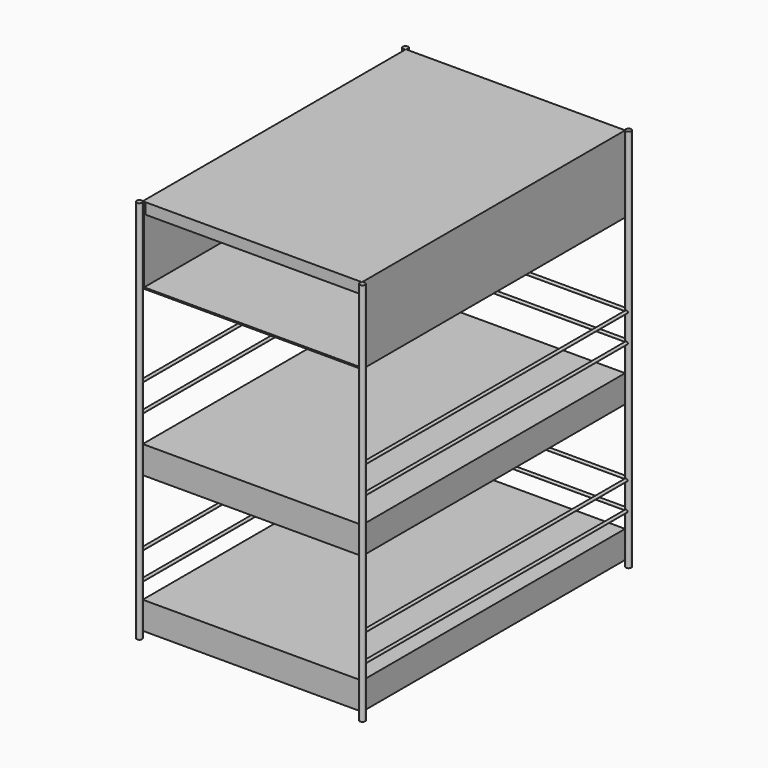
from build123d import *

# Parameters (mm, degrees)
F0_W      = 400
F0_H      = 140
F1_DEPTH  = 600
F0_H_2    = 50
F2_R      = 5
F3_DEPTH  = 701.04
F5_T      = -2.54
F4_W      = 390
F4_H      = 20
F6_DEPTH  = 25.4
F8_R      = 2.5
F9_DEPTH  = 607.822
F11_R     = 2.5
F12_DEPTH = 407.162


with BuildPart() as f1:
    # F0 (on Front) → F1 (new body)
    with BuildSketch(Plane.XZ):
        with Locations((0, 345)):
            Rectangle(F0_W, F0_H)
    extrude(amount=-F1_DEPTH)

    # F5
    f5_openings = [f1.faces().sort_by_distance(p)[0] for p in [
        (0, 0, 345),
    ]]
    offset(amount=F5_T, openings=f5_openings)

    # F4 (on face) → F6 (join)
    with BuildSketch(Plane.XZ):
        with Locations((0, 405)):
            Rectangle(F4_W, F4_H)
    extrude(amount=-F6_DEPTH)


with BuildPart() as f1b:
    # F0 (on Front) → F1, piece 2 (new body)
    with BuildSketch(Plane.XZ):
        Rectangle(F0_W, F0_H_2)
    extrude(amount=-F1_DEPTH)


with BuildPart() as f1c:
    # F0 (on Front) → F1, piece 3 (new body)
    with BuildSketch(Plane.XZ):
        with Locations((0, -250)):
            Rectangle(F0_W, F0_H_2)
    extrude(amount=-F1_DEPTH)


with BuildPart() as f3:
    # F2 (on face) → F3 (new body)
    with BuildSketch(Plane.XY.offset(415)):
        with Locations((203.5355339059, -3.5355339059)):
            Circle(F2_R)
    extrude(amount=-F3_DEPTH)


with BuildPart() as f3b:
    # F2 (on face) → F3, piece 2 (new body)
    with BuildSketch(Plane.XY.offset(415)):
        with Locations((203.5355339059, 603.5355339059)):
            Circle(F2_R)
    extrude(amount=-F3_DEPTH)


with BuildPart() as f3c:
    # F2 (on face) → F3, piece 3 (new body)
    with BuildSketch(Plane.XY.offset(415)):
        with Locations((-203.5355339059, 603.5355339059)):
            Circle(F2_R)
    extrude(amount=-F3_DEPTH)


with BuildPart() as f3d:
    # F2 (on face) → F3, piece 4 (new body)
    with BuildSketch(Plane.XY.offset(415)):
        with Locations((-202.7795129572, -4.156237207)):
            Circle(F2_R)
    extrude(amount=-F3_DEPTH)


with BuildPart() as f9:
    # F8 (on face) → F9 (new body)
    with BuildSketch(Plane(origin=(0, 603.5355339059, 0), x_dir=(-1, 0, 0), z_dir=(0, 1, 0))):
        with Locations((202.33258605, 125)):
            Circle(F8_R)
    extrude(amount=-F9_DEPTH)


with BuildPart() as f9b:
    # F8 (on face) → F9, piece 2 (new body)
    with BuildSketch(Plane(origin=(0, 603.5355339059, 0), x_dir=(-1, 0, 0), z_dir=(0, 1, 0))):
        with Locations((202.33258605, 75)):
            Circle(F8_R)
    extrude(amount=-F9_DEPTH)


with BuildPart() as f9c:
    # F8 (on face) → F9, piece 3 (new body)
    with BuildSketch(Plane(origin=(0, 603.5355339059, 0), x_dir=(-1, 0, 0), z_dir=(0, 1, 0))):
        with Locations((-203.3087313175, 125)):
            Circle(F8_R)
    extrude(amount=-F9_DEPTH)


with BuildPart() as f9d:
    # F8 (on face) → F9, piece 4 (new body)
    with BuildSketch(Plane(origin=(0, 603.5355339059, 0), x_dir=(-1, 0, 0), z_dir=(0, 1, 0))):
        with Locations((-203.3087313175, 75)):
            Circle(F8_R)
    extrude(amount=-F9_DEPTH)


with BuildPart() as f9e:
    # F8 (on face) → F9, piece 5 (new body)
    with BuildSketch(Plane(origin=(0, 603.5355339059, 0), x_dir=(-1, 0, 0), z_dir=(0, 1, 0))):
        with Locations((202.33258605, -145)):
            Circle(F8_R)
    extrude(amount=-F9_DEPTH)


with BuildPart() as f9f:
    # F8 (on face) → F9, piece 6 (new body)
    with BuildSketch(Plane(origin=(0, 603.5355339059, 0), x_dir=(-1, 0, 0), z_dir=(0, 1, 0))):
        with Locations((202.33258605, -195)):
            Circle(F8_R)
    extrude(amount=-F9_DEPTH)


with BuildPart() as f9g:
    # F8 (on face) → F9, piece 7 (new body)
    with BuildSketch(Plane(origin=(0, 603.5355339059, 0), x_dir=(-1, 0, 0), z_dir=(0, 1, 0))):
        with Locations((-202.9743790627, -145)):
            Circle(F8_R)
    extrude(amount=-F9_DEPTH)


with BuildPart() as f9h:
    # F8 (on face) → F9, piece 8 (new body)
    with BuildSketch(Plane(origin=(0, 603.5355339059, 0), x_dir=(-1, 0, 0), z_dir=(0, 1, 0))):
        with Locations((-202.9743790627, -195)):
            Circle(F8_R)
    extrude(amount=-F9_DEPTH)


with BuildPart() as f12:
    # F11 (on face) → F12 (new body)
    with BuildSketch(Plane.YZ.offset(-203.5355339059)):
        with Locations((604.149222374, 124.5824322104)):
            Circle(F11_R)
    extrude(amount=F12_DEPTH)


with BuildPart() as f12b:
    # F11 (on face) → F12, piece 2 (new body)
    with BuildSketch(Plane.YZ.offset(-203.5355339059)):
        with Locations((604.149222374, 75.2380788326)):
            Circle(F11_R)
    extrude(amount=F12_DEPTH)


with BuildPart() as f12c:
    # F11 (on face) → F12, piece 3 (new body)
    with BuildSketch(Plane.YZ.offset(-203.5355339059)):
        with Locations((604.1088700294, -145.0297236443)):
            Circle(F11_R)
    extrude(amount=F12_DEPTH)


with BuildPart() as f12d:
    # F11 (on face) → F12, piece 4 (new body)
    with BuildSketch(Plane.YZ.offset(-203.5355339059)):
        with Locations((603.9840579033, -195.2335387468)):
            Circle(F11_R)
    extrude(amount=F12_DEPTH)


solid = Compound([f1.part, f1b.part, f1c.part, f3.part, f3b.part, f3c.part, f3d.part, f9.part, f9b.part, f9c.part, f9d.part, f9e.part, f9f.part, f9g.part, f9h.part, f12.part, f12b.part, f12c.part, f12d.part])
